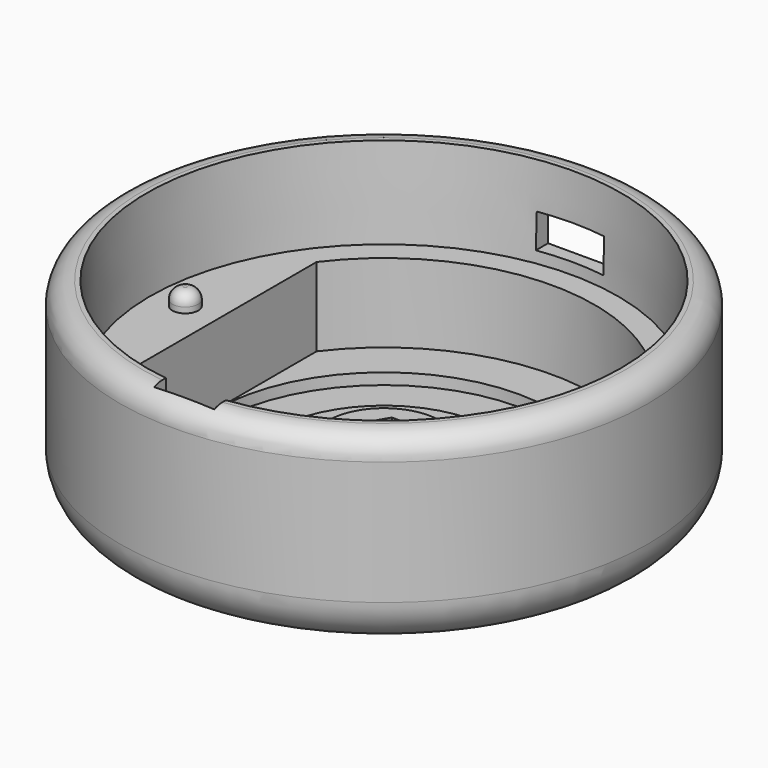
from build123d import *

# Parameters (mm, degrees)
F0_R      = 29.845
F1_DEPTH  = 21.59
F2_R      = 26.797
F3_DEPTH  = 10.16
F3_TAPER  = 2
F4_R      = 23.8125
F5_DEPTH  = 8.89
F6_R      = 6.35
F7_DEPTH  = 3.048
F8_R      = 2.54
F9_DEPTH  = 25.4
F12_DEPTH = 3.302
F13_R     = 5.08
F14_R     = 2.54
F15_R     = 19.05
F15_R_2   = 12.7
F16_DEPTH = 1.27
F18_DEPTH = 8.89
F19_R     = 1.4605
F20_DEPTH = 1.905
F21_R     = 1.27
F22_W     = 7.62
F22_H     = 3.81
F23_DEPTH = 36.576
F25_DEPTH = 16.51
F27_DEPTH = 19.0510001
F29_W     = 11.43
F29_H     = 7.62
F30_DEPTH = 3.81


with BuildPart() as f1:
    # F0 (on Top) → F1 (new body)
    with BuildSketch(Plane.XY):
        Circle(F0_R)
    extrude(amount=F1_DEPTH)

    # F2 (on face) → F3 (cut)
    with BuildSketch(Plane.XY.offset(21.59)):
        Circle(F2_R)
    extrude(amount=-F3_DEPTH, taper=F3_TAPER, mode=Mode.SUBTRACT)

    # F4 (on face) → F5 (cut)
    with BuildSketch(Plane.XY.offset(11.43)):
        Circle(F4_R)
    extrude(amount=-F5_DEPTH, mode=Mode.SUBTRACT)

    # F6 (on face) → F7 (join)
    with BuildSketch(Plane.XY.offset(2.54)):
        Circle(F6_R)
    extrude(amount=F7_DEPTH)

    # F8 (on face) → F9 (cut)
    with BuildSketch(Plane.XY.offset(5.588)):
        Circle(F8_R)
    extrude(amount=-F9_DEPTH, mode=Mode.SUBTRACT)

    # F11 (on offset) → F12 (cut)
    with BuildSketch(Plane.XY.offset(5.588)):
        Polygon((-2.3096897519, -4.0005), (2.3096897519, -4.0005), (4.6193795038, 0), (2.3096897519, 4.0005), (-2.3096897519, 4.0005), (-4.6193795038, 0), align=None)
    extrude(amount=-F12_DEPTH, mode=Mode.SUBTRACT)

    # F13
    f13_edges = [f1.edges().sort_by_distance(p)[0] for p in [
        (-29.845, 0, 0),
    ]]
    fillet(f13_edges, radius=F13_R)

    # F14
    f14_edges = [f1.edges().sort_by_distance(p)[0] for p in [
        (-29.845, 0, 21.59),
    ]]
    fillet(f14_edges, radius=F14_R)

    # F15 (on face) → F16 (cut)
    with BuildSketch(Plane.XY.offset(2.54)):
        Circle(F15_R)
        Circle(F15_R_2, mode=Mode.SUBTRACT)
    extrude(amount=-F16_DEPTH, mode=Mode.SUBTRACT)

    # F17 (on face) → F18 (join, through all)
    with BuildSketch(Plane.XY.offset(2.54)):
        with BuildLine():
            Line((-19.05, 0), (-19.05, 14.2875))
            ThreePointArc((-19.05, 14.2875), (-23.8125, 0), (-19.05, -14.2875))
            Line((-19.05, -14.2875), (-19.05, 0))
        make_face()
        with BuildLine():
            ThreePointArc((23.8125, 0), (22.5905210348, 7.5301736783), (19.05, 14.2875))
            Line((19.05, 14.2875), (19.05, 0))
            Line((19.05, 0), (19.05, -14.2875))
            ThreePointArc((19.05, -14.2875), (22.5905210348, -7.5301736783), (23.8125, 0))
        make_face()
    extrude(amount=F18_DEPTH)

    # F19 (on face) → F20 (join)
    with BuildSketch(Plane.XY.offset(11.43)):
        with Locations((-22.86, 0.508)):
            Circle(F19_R)
        with Locations((22.86, 0.508)):
            Circle(F19_R)
    extrude(amount=F20_DEPTH)

    # F21
    f21_edges = [f1.edges().sort_by_distance(p)[0] for p in [
        (-24.3205, 0.508, 13.335),
        (21.3995, 0.508, 13.335),
    ]]
    fillet(f21_edges, radius=F21_R)

    # F22 (on Front) → F23 (cut)
    with BuildSketch(Plane.XZ):
        with Locations((0, 14.605)):
            Rectangle(F22_W, F22_H)
    extrude(amount=-F23_DEPTH, mode=Mode.SUBTRACT)

    # F24 (on face) → F25 (cut)
    with BuildSketch(Plane.XY.offset(21.59)):
        with BuildLine():
            ThreePointArc((-3.39725, -26.5807806777), (0, -26.797), (3.39725, -26.5807806777))
            Line((3.39725, -26.5807806777), (3.39725, -23.129734925))
            Line((3.39725, -23.129734925), (-3.39725, -23.129734925))
            Line((-3.39725, -23.129734925), (-3.39725, -26.5807806777))
        make_face()
        with BuildLine():
            Line((-3.39725, -28.209734925), (3.39725, -28.209734925))
            Line((3.39725, -28.209734925), (3.39725, -27.0928351679))
            ThreePointArc((3.39725, -27.0928351679), (0, -27.305), (-3.39725, -27.0928351679))
            Line((-3.39725, -27.0928351679), (-3.39725, -28.209734925))
        make_face()
        with BuildLine():
            ThreePointArc((-3.39725, -27.0928351679), (0, -27.305), (3.39725, -27.0928351679))
            Line((3.39725, -27.0928351679), (3.39725, -26.5807806777))
            ThreePointArc((3.39725, -26.5807806777), (0, -26.797), (-3.39725, -26.5807806777))
            Line((-3.39725, -26.5807806777), (-3.39725, -27.0928351679))
        make_face()
    extrude(amount=-F25_DEPTH, mode=Mode.SUBTRACT)

    # F26 (on face) → F27 (cut, through all)
    with BuildSketch(Plane.XY.offset(2.54)):
        with BuildLine():
            ThreePointArc((19.05, -14.2875), (0, -23.8125), (-19.05, -14.2875))
            Line((-19.05, -14.2875), (-19.05, -16.3165347501))
            ThreePointArc((-19.05, -16.3165347501), (0, -25.0825), (19.05, -16.3165347501))
            Line((19.05, -16.3165347501), (19.05, -14.2875))
        make_face()
    extrude(amount=F27_DEPTH, mode=Mode.SUBTRACT)

    # F29 (on offset) → F30 (cut)
    with BuildSketch(Plane.XZ.offset(-31.75)):
        with Locations((0, 14.605)):
            Rectangle(F29_W, F29_H)
    extrude(amount=F30_DEPTH, mode=Mode.SUBTRACT)


solid = f1.part
